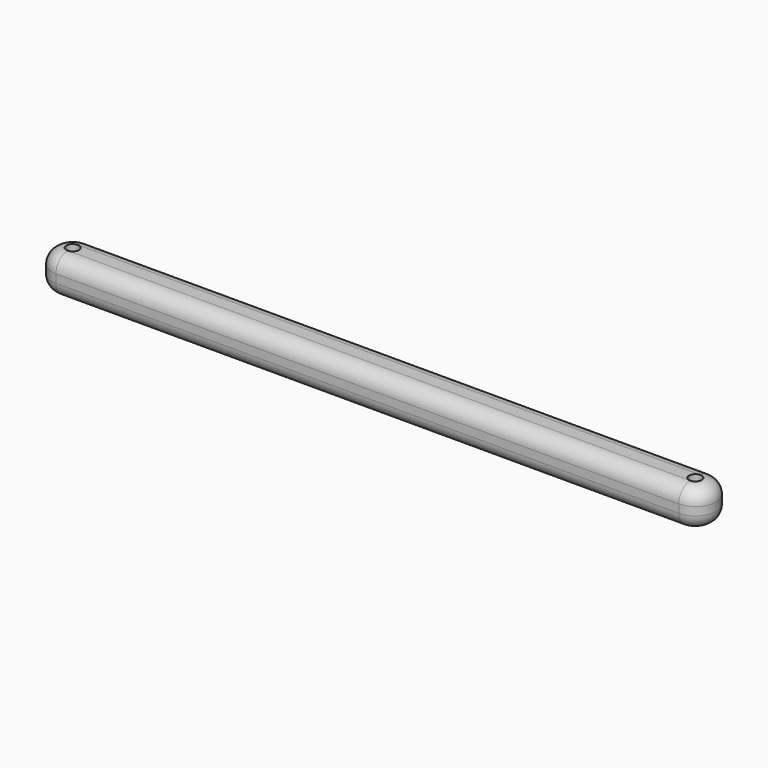
from build123d import *

# Parameters (mm, degrees)
F0_R     = 1.5
F1_DEPTH = 9
F2_R     = 3.49999


# Not quite as in the source:
# - a fillet or chamfer is up to 0.001 mm smaller than in the source, because OpenCascade refuses the exact size


with BuildPart() as f1:
    # F0 (on Top) → F1 (new body)
    with BuildSketch(Plane.XY):
        with BuildLine():
            Line((150, 5), (0, 5))
            ThreePointArc((0, 5), (-5, 0), (0, -5))
            Line((0, -5), (150, -5))
            ThreePointArc((150, -5), (155, 0), (150, 5))
        make_face()
        Circle(F0_R, mode=Mode.SUBTRACT)
        with Locations((150, 0)):
            Circle(F0_R, mode=Mode.SUBTRACT)
    extrude(amount=F1_DEPTH)

    # F2 (radius 3.5 in the source; OpenCascade refuses exactly that, so slightly less here)
    f2_edges = [f1.edges().sort_by_distance(p)[0] for p in [
        (75, 5, 9),
        (75, -5, 0),
    ]]
    fillet(f2_edges, radius=F2_R)


solid = f1.part
